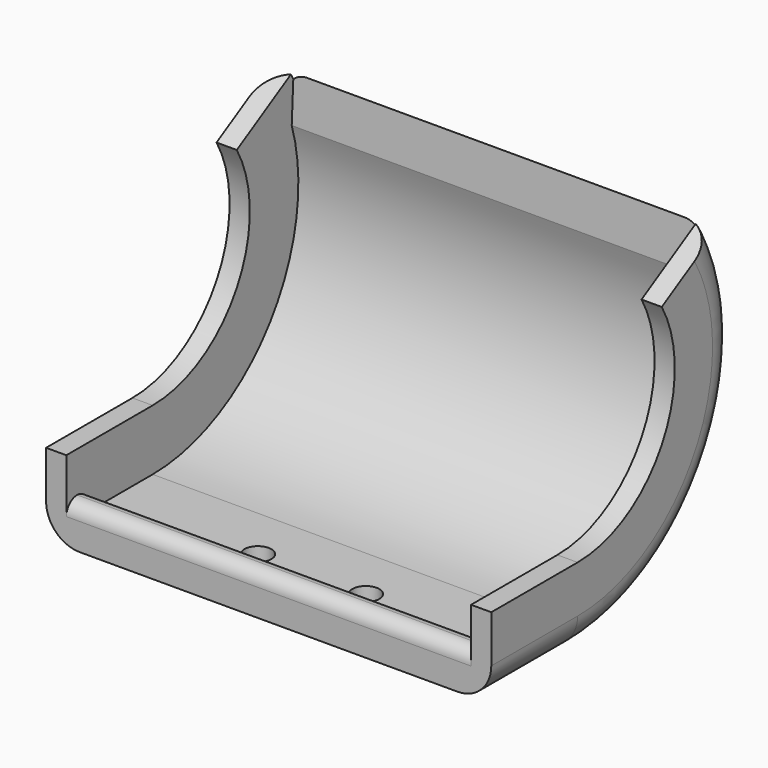
from build123d import *

# Parameters (mm, degrees)
F1_ANGLE    = 120
F2_T1_DEPTH = 60
F3_T2_ANGLE = 167.7805884334
F3_T4_ANGLE = 167.7805884334
F4_DEPTH    = 16
F5_R        = 2
F6_DEPTH    = 3.0010001
F5_W        = 60
F5_H        = 4
F7_DEPTH    = 3
F8_R        = 1.99999


# Not quite as in the source:
# - a fillet or chamfer that OpenCascade refuses, or shapes differently, is made with other operations: its cross-section is extruded or revolved along the edge and cut away or added
# - a fillet or chamfer is up to 0.001 mm smaller than in the source, because OpenCascade refuses the exact size


with BuildPart() as f1:
    # F0 (on Front) → F1 (revolve)
    with BuildSketch(Plane.XZ):
        Polygon((-33, 12), (-33, 0), (33, 0), (33, 12), (30, 12), (30, 3), (-30, 3), (-30, 12), align=None)
    revolve(axis=Axis((7.0132222027, 0, 30), (1, 0, 0)), revolution_arc=F1_ANGLE)

    # F2: chamfer of 3.9 x 6.7549981495 on 1 edges, made by hand

    # F2_s2 → F2_t1 (cut)
    with BuildSketch(Plane.YZ.offset(-30)):
        with BuildLine():
            Line((25.7683341911, 38.0618207012), (26.1129278328, 45.0763059136))
            Line((26.1129278328, 45.0763059136), (23.3826859022, 43.5))
            ThreePointArc((23.3826859022, 43.5), (24.7742012809, 40.7349406562), (25.7683341911, 38.0618207012))
        make_face()
    extrude(amount=F2_T1_DEPTH, mode=Mode.SUBTRACT)

    # F3: fillet of radius 5 on 2 edges, made by hand

    # F3_s1 → F3_t2 (revolve, cut)
    with BuildSketch(Plane(origin=(0, -11.1086546654, 4.9204270168), x_dir=(1, 0, 0), z_dir=(0, -0.9143225722, 0.4049867083))):
        with BuildLine():
            ThreePointArc((28, -2.5703228328), (31.5355339059, -1.1058567387), (33, 2.4296771672))
            Line((33, 2.4296771672), (33, -2.5703228328))
            Line((33, -2.5703228328), (28, -2.5703228328))
        make_face()
    revolve(axis=Axis((33, 0, 30), (1, 0, 0)), revolution_arc=F3_T2_ANGLE, mode=Mode.SUBTRACT)

    # F3_s3 → F3_t4 (revolve, cut)
    with BuildSketch(Plane(origin=(0, -11.1086546654, 4.9204270168), x_dir=(1, 0, 0), z_dir=(0, -0.9143225722, 0.4049867083))):
        with BuildLine():
            ThreePointArc((-33, 2.4296771672), (-31.5355339059, -1.1058567387), (-28, -2.5703228328))
            Line((-28, -2.5703228328), (-33, -2.5703228328))
            Line((-33, -2.5703228328), (-33, 2.4296771672))
        make_face()
    revolve(axis=Axis((-33, 0, 30), (1, 0, 0)), revolution_arc=F3_T4_ANGLE, mode=Mode.SUBTRACT)

    # F4 (add): a face of the model
    f4_faces = [f1.faces().sort_by_distance(p)[0] for p in [
        (0, 0, 2.8599348039),
    ]]
    extrude(f4_faces, amount=F4_DEPTH)

    # F5 (on face) → F6 (cut, through all)
    with BuildSketch(Plane.XY.offset(3)):
        with Locations((-8, -8)):
            Circle(F5_R)
        with Locations((8, -8)):
            Circle(F5_R)
    extrude(amount=-F6_DEPTH, mode=Mode.SUBTRACT)

    # F5 (on face) → F7 (join)
    with BuildSketch(Plane.XY.offset(3)):
        with Locations((0, -14)):
            Rectangle(F5_W, F5_H)
    extrude(amount=F7_DEPTH)

    # F8 (radius 2 in the source; OpenCascade refuses exactly that, so slightly less here)
    f8_edges = [f1.edges().sort_by_distance(p)[0] for p in [
        (0, -16, 6),
        (0, -12, 6),
    ]]
    fillet(f8_edges, radius=F8_R)


solid = f1.part
